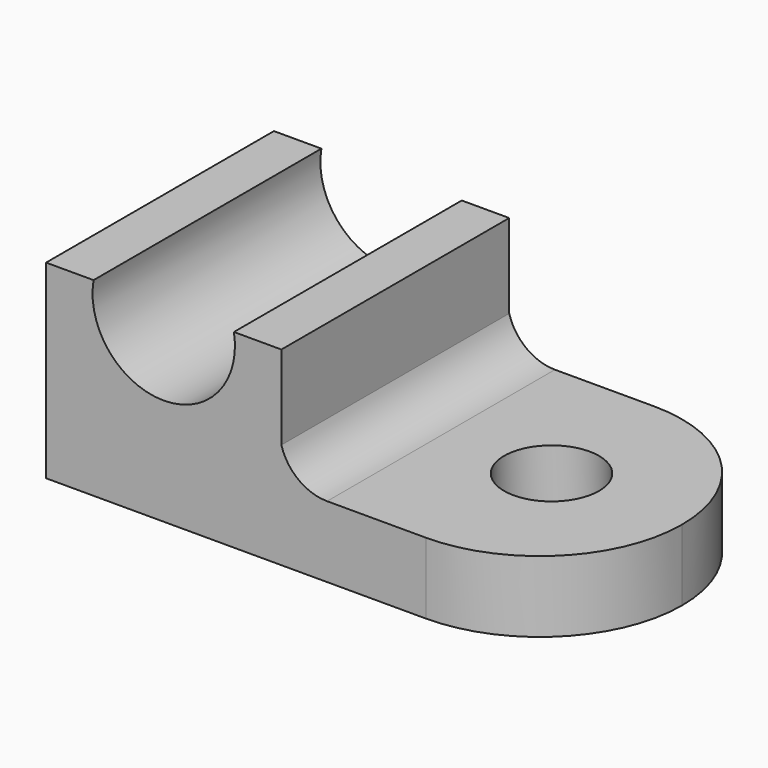
from build123d import *

# Parameters (mm, degrees)
F1_DEPTH = 76.2
F2_R     = 38.09999
F3_R     = 12.7
F4_DEPTH = 50.8
F5_DEPTH = 25.4


# Not quite as in the source:
# - a fillet or chamfer is up to 0.001 mm smaller than in the source, because OpenCascade refuses the exact size


with BuildPart() as f1:
    # F0 (on Front) → F1 (new body)
    with BuildSketch(Plane.XZ):
        with BuildLine():
            Line((-50.2547219646, 33.020831282), (-62.9547219646, 33.020831282))
            Line((-62.9547219646, 33.020831282), (-62.9547219646, -17.779168718))
            Line((-62.9547219646, -17.779168718), (76.7452780354, -17.779168718))
            Line((76.7452780354, -17.779168718), (76.7452780354, 1.270831282))
            Line((76.7452780354, 1.270831282), (12.2243361415, 1.270831282))
            ThreePointArc((12.2243361415, 1.270831282), (4.5574789786, 3.8461435711), (0, 10.5276342357))
            Line((0, 10.5276342357), (0, 33.020831282))
            Line((0, 33.020831282), (-12.7, 33.020831282))
            ThreePointArc((-12.7, 33.020831282), (-31.4773609823, 10.7594118855), (-50.2547219646, 33.020831282))
        make_face()
    extrude(amount=F1_DEPTH)

    # F2 (radius 38.1 in the source; OpenCascade refuses exactly that, so slightly less here)
    f2_edges = [f1.edges().sort_by_distance(p)[0] for p in [
        (76.745278, -76.2, -8.254169),
        (76.745278, 0, -8.254169),
    ]]
    fillet(f2_edges, radius=F2_R)

    # F3 (on Top) → F4 (cut)
    with BuildSketch(Plane.XY):
        with Locations((40.9884415567, -37.0847843587)):
            Circle(F3_R)
    extrude(amount=F4_DEPTH, mode=Mode.SUBTRACT)

    # F5 (cut): a face of the model
    f5_faces = [f1.faces().sort_by_distance(p)[0] for p in [
        (40.9884415567, -37.0847843587, 0),
    ]]
    extrude(f5_faces, amount=-F5_DEPTH, mode=Mode.SUBTRACT)


solid = f1.part
